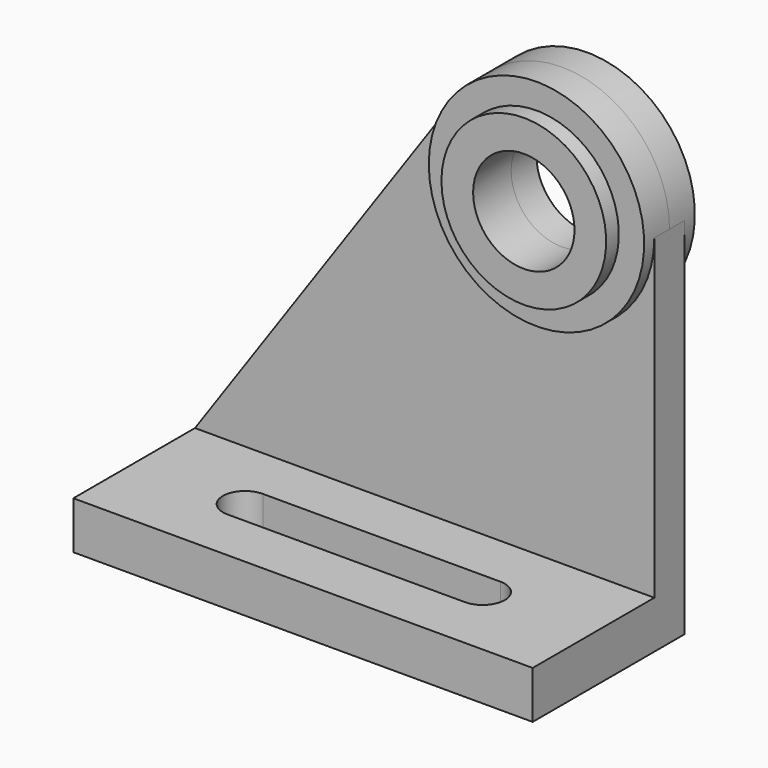
from build123d import *

# Parameters (mm, degrees)
F0_W     = 145
F0_H     = 12
F1_DEPTH = 15
F4_DEPTH = 12
F6_R     = 26
F6_R_2   = 16
F7_DEPTH = 10
F8_DEPTH = 10
F9_DEPTH = 15


with BuildPart() as f1:
    # F0 (on Top) → F1 (new body)
    with BuildSketch(Plane.XY):
        with Locations((0, 30)):
            Rectangle(F0_W, F0_H)
        Polygon((-72.5, 24), (-72.5, 0), (-72.5, -24), (-37.5, -24), (37.5, -24), (72.5, -24), (72.5, 0), (72.5, 24), align=None)
        with BuildLine():
            Line((37.5, -7), (-37.5, -7))
            ThreePointArc((-37.5, -7), (-44.5, 0), (-37.5, 7))
            Line((-37.5, 7), (37.5, 7))
            ThreePointArc((37.5, 7), (44.5, 0), (37.5, -7))
        make_face(mode=Mode.SUBTRACT)
    extrude(amount=-F1_DEPTH)

    # F3 (on offset) → F4 (join)
    with BuildSketch(Plane(origin=(0, 36, 0), x_dir=(-1, 0, 0), z_dir=(0, 1, 0))):
        with BuildLine():
            ThreePointArc((-10.5910955607, 119.4188839277), (-6.0584930148, 110.1758844594), (-4.5, 100))
            ThreePointArc((-4.5, 100), (-38.5, 66), (-72.5, 100))
            Line((-72.5, 100), (-72.5, 0))
            Line((-72.5, 0), (72.5, 0))
            Line((72.5, 0), (-10.5910955607, 119.4188839277))
        make_face()
    extrude(amount=-F4_DEPTH)

    # F6 (on offset) → F7 (join)
    with BuildSketch(Plane(origin=(0, 30, 0), x_dir=(-1, 0, 0), z_dir=(0, 1, 0))):
        with BuildLine():
            ThreePointArc((-72.5, 100), (-38.5, 66), (-4.5, 100))
            ThreePointArc((-4.5, 100), (-38.5, 134), (-72.5, 100))
        make_face()
        with Locations((-38.5, 100)):
            Circle(F6_R, mode=Mode.SUBTRACT)
        with Locations((-38.5, 100)):
            Circle(F6_R)
        with Locations((-38.5, 100)):
            Circle(F6_R_2, mode=Mode.SUBTRACT)
    extrude(amount=F7_DEPTH)

    # F6 (on offset) → F8 (join)
    with BuildSketch(Plane(origin=(0, 30, 0), x_dir=(-1, 0, 0), z_dir=(0, 1, 0))):
        with BuildLine():
            ThreePointArc((-72.5, 100), (-38.5, 66), (-4.5, 100))
            ThreePointArc((-4.5, 100), (-38.5, 134), (-72.5, 100))
        make_face()
        with Locations((-38.5, 100)):
            Circle(F6_R, mode=Mode.SUBTRACT)
    extrude(amount=-F8_DEPTH)

    # F6 (on offset) → F9 (join)
    with BuildSketch(Plane(origin=(0, 30, 0), x_dir=(-1, 0, 0), z_dir=(0, 1, 0))):
        with Locations((-38.5, 100)):
            Circle(F6_R)
        with Locations((-38.5, 100)):
            Circle(F6_R_2, mode=Mode.SUBTRACT)
    extrude(amount=-F9_DEPTH)


solid = f1.part
